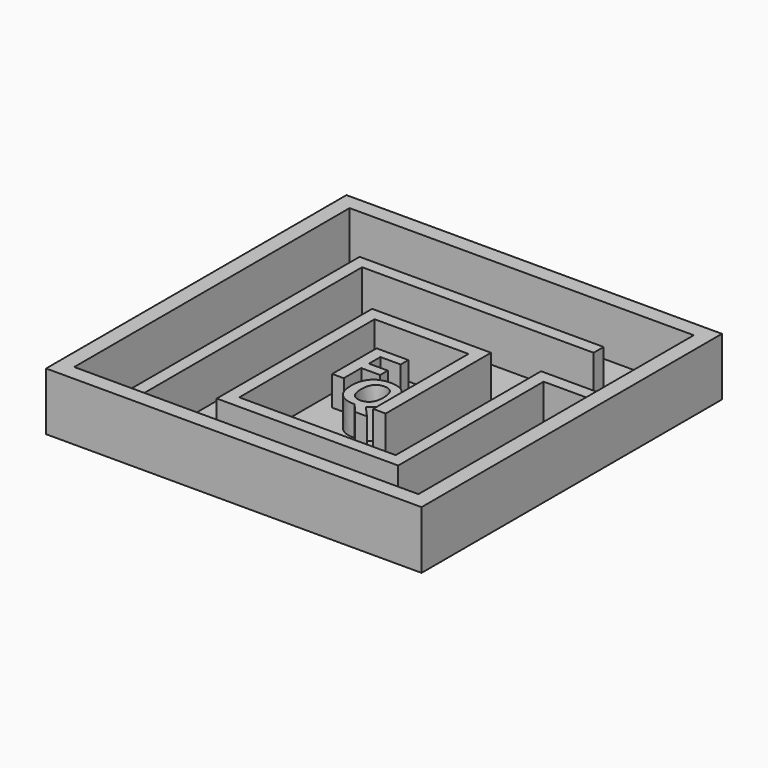
from build123d import *

# Parameters (mm, degrees)
F0_W           = 38.1
F0_H           = 38.1
F1_DEPTH       = 0.79375
F2_W           = 38.1
F2_H           = 38.1
F2_W_2         = 34.925
F2_H_2         = 34.925
F3_DEPTH       = 5.08
F6_DEPTH       = 4.445
F7_DEPTH       = 4.445
F5_R           = 1.27
F8_DEPTH       = 0.396875
F9_TEXT_SIZE   = 7.8825159324
F9_TEXT_SIZE_2 = 6.3289857894
F10_DEPTH      = 3.81


# Not quite as in the source:
# - Text() gives the source's letters only with a copy of the font that has no kerning and outlines rounded to 1/6400 em; it was checked with that copy


with BuildPart() as f1:
    # F0 (on Top) → F1 (new body)
    with BuildSketch(Plane.XY):
        with Locations((12.0160095394, -7.8415322932)):
            Rectangle(F0_W, F0_H)
    extrude(amount=F1_DEPTH)

    # F2 (on face) → F3 (join)
    with BuildSketch(Plane.XY.offset(0.79375)):
        with Locations((12.0160095394, -7.8415322932)):
            Rectangle(F2_W, F2_H)
        with Locations((12.0160095394, -7.8415322932)):
            Rectangle(F2_W_2, F2_H_2, mode=Mode.SUBTRACT)
    extrude(amount=F3_DEPTH)

    # F4 (on face) → F6 (join)
    with BuildSketch(Plane.XY.offset(0.79375)):
        Polygon((0.9035095394, 4.5409677068), (-0.3664904606, 4.5409677068), (-0.3664904606, -25.3040322932), (0.9035095394, -25.3040322932), (0.9035095394, -14.0136955306), (0.9035095394, -12.7436955306), (0.9035095394, 3.2709677068), (24.3985095394, 3.2709677068), (24.3985095394, 4.5409677068), align=None)
    extrude(amount=F6_DEPTH)

    # F4 (on face) → F7 (join)
    with BuildSketch(Plane.XY.offset(0.79375)):
        Polygon((24.3985095394, -3.0790322932), (29.4785095394, -3.0790322932), (29.4785095394, -1.8090322932), (23.1285095394, -1.8090322932), (23.1285095394, -3.0790322932), (23.1285095394, -20.2492586184), (7.2535095394, -20.2492586184), (7.2535095394, -14.0136955306), (7.2535095394, -3.0790322932), (10.3655606508, -3.0790322932), (11.2058715895, -3.0790322932), (16.7785095394, -3.0790322932), (16.7785095394, -15.1692586184), (18.0485095394, -15.1692586184), (18.0485095394, -3.0790322932), (18.0485095394, -1.8090322932), (13.6035095394, -1.8090322932), (12.3335095394, -1.8090322932), (5.9835095394, -1.8090322932), (5.9835095394, -3.0790322932), (5.9835095394, -12.7436955306), (5.9835095394, -14.0136955306), (5.9835095394, -21.5192586184), (7.2535095394, -21.5192586184), (23.1285095394, -21.5192586184), (24.3985095394, -21.5192586184), align=None)
    extrude(amount=F7_DEPTH)

    # F5 (on face) → F8 (cut)
    with BuildSketch(Plane.XY.offset(0.79375)):
        with Locations((-2.9306163924, -22.5373676107)):
            Circle(F5_R)
        with Locations((11.9807126466, -16.5028627962)):
            Circle(F5_R)
    extrude(amount=-F8_DEPTH, mode=Mode.SUBTRACT)

    # F9 (on Top) → F10 (join)
    with BuildSketch(Plane.XY):
        with Locations((8.0675656367, -10.3637021397)):
            Text('F', F9_TEXT_SIZE, font='Open Sans', font_style=FontStyle.BOLD, text_align=(TextAlign.LEFT, TextAlign.BOTTOM))
        with Locations((10.8296088874, -13.2497054583)):
            Text('Q', F9_TEXT_SIZE_2, font='Open Sans', font_style=FontStyle.BOLD, text_align=(TextAlign.LEFT, TextAlign.BOTTOM))
    extrude(amount=F10_DEPTH)


solid = f1.part
